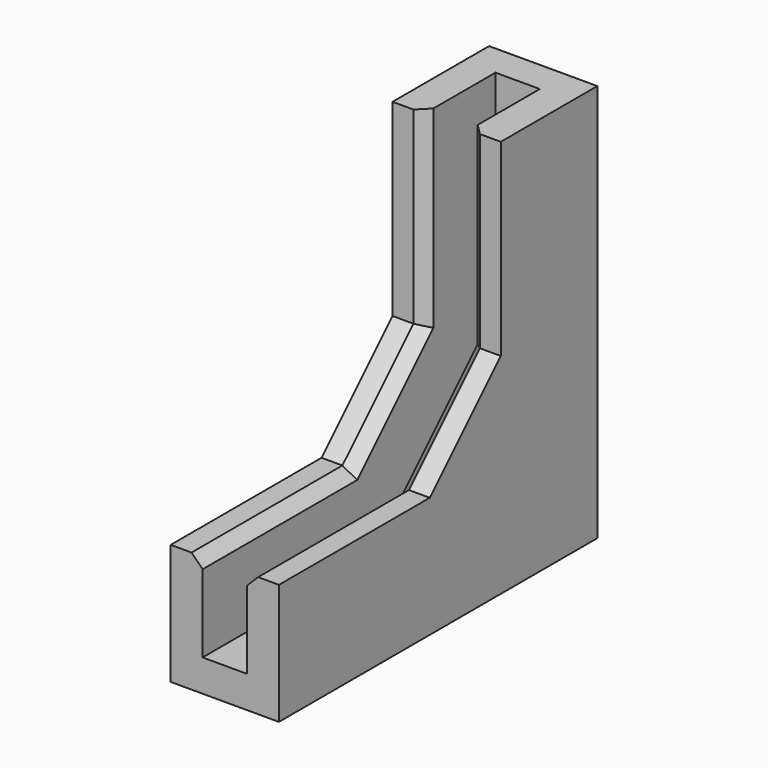
from build123d import *

# Parameters (mm, degrees)
F3_SIZE = 8
F4_SIZE = 1


with BuildPart() as f2:
    # F2: sweep along a path in F0
    with BuildLine(Plane.YZ) as f2_path:
        Line((-25, 0), (0, 0))
        Line((0, 0), (0, 25))
    # F1 (on Front) → F2 (sweep)
    with BuildSketch(Plane.XZ):
        Polygon((-2, -8), (-2, 0), (-4.88, 0), (-4.88, -10.88), (4.88, -10.88), (4.88, 0), (2, 0), (2, -8), align=None)
    sweep(path=f2_path.line, transition=Transition.RIGHT)

    # F3
    f3_edges = [f2.edges().sort_by_distance(p)[0] for p in [
        (-3.44, 0, 0),
        (3.44, 0, 0),
    ]]
    chamfer(f3_edges, length=F3_SIZE)

    # F4
    f4_edges = [f2.edges().sort_by_distance(p)[0] for p in [
        (-2, -16.5, 0),
        (-2, 0, 16.5),
        (2, 0, 16.5),
        (2, -16.5, 0),
        (-2, -4, 4),
        (2, -4, 4),
    ]]
    chamfer(f4_edges, length=F4_SIZE)


solid = f2.part
